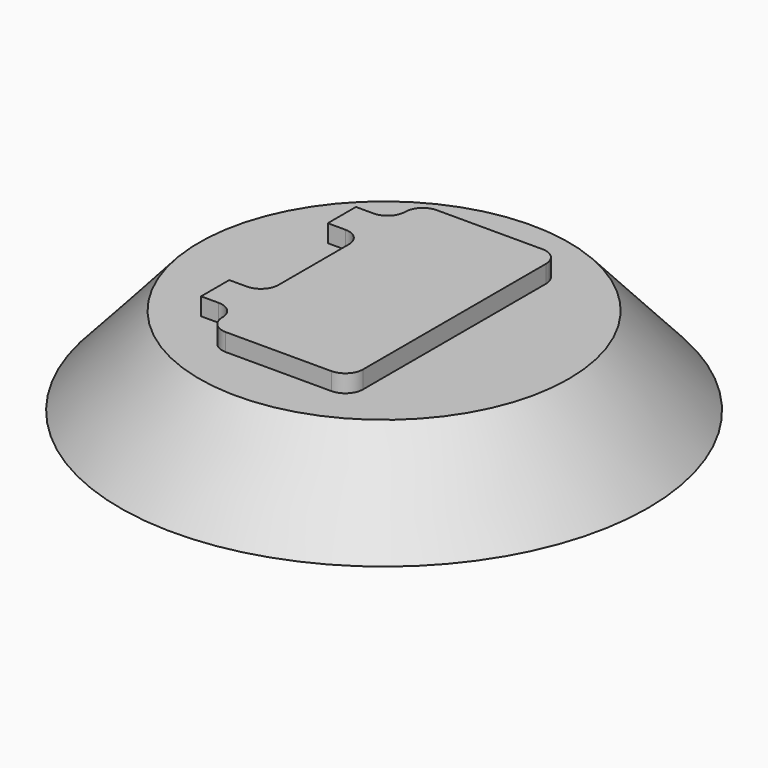
from build123d import *

# Parameters (mm, degrees)
F0_R     = 15
F2_R     = 10.5
F5_DEPTH = 1
F6_R     = 0.99999


# Not quite as in the source:
# - a fillet or chamfer is up to 0.001 mm smaller than in the source, because OpenCascade refuses the exact size


with BuildPart() as f3:
    # F0 (on Top) → F3 section 0
    with BuildSketch(Plane.XY):
        Circle(F0_R)
    # F2 (on offset) → F3 section 1
    with BuildSketch(Plane.XY.offset(5)):
        Circle(F2_R)
    loft()

    # F4 (on face) → F5 (join)
    with BuildSketch(Plane.XY.offset(5)):
        Polygon((-4, -5.5), (-4, -7.5), (4, -7.5), (4, 7.5), (-4, 7.5), (-4, 5.5), (-6, 5.5), (-6, 3.5), (-4, 3.5), (-4, -3.5), (-6, -3.5), (-6, -5.5), align=None)
    extrude(amount=F5_DEPTH)

    # F6 (radius 1 in the source; OpenCascade refuses exactly that, so slightly less here)
    f6_edges = [f3.edges().sort_by_distance(p)[0] for p in [
        (-4, -7.5, 5.5),
        (4, -7.5, 5.5),
        (4, 7.5, 5.5),
        (-4, 7.5, 5.5),
        (-4, -5.5, 5.5),
        (-4, 3.5, 5.5),
        (-4, -3.5, 5.5),
        (-4, 5.5, 5.5),
    ]]
    fillet(f6_edges, radius=F6_R)


solid = f3.part
